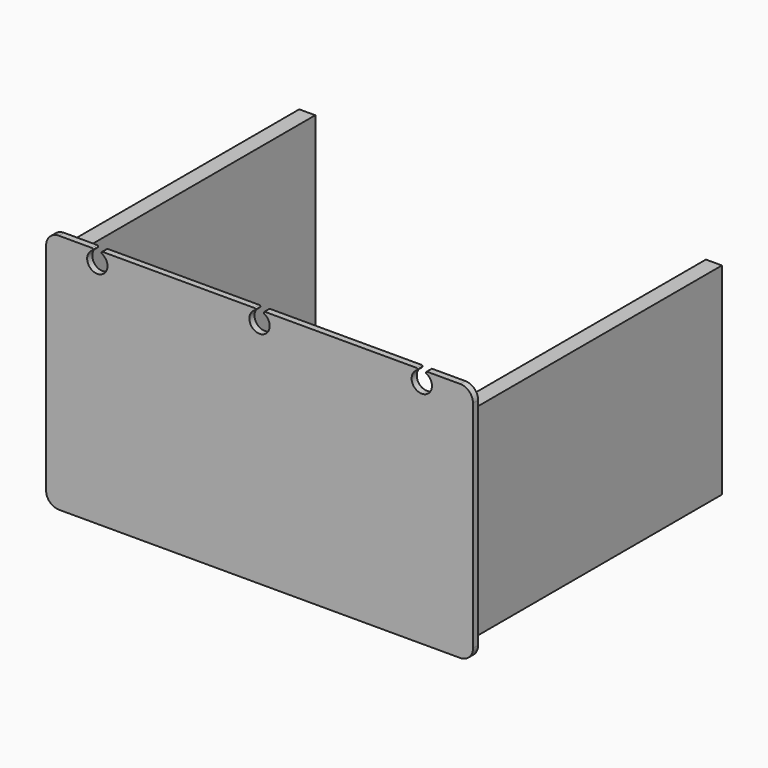
from build123d import *

# Parameters (mm, degrees)
F0_W     = 47.625
F0_H     = 600.075
F1_DEPTH = 914.4
F2_W     = 47.625
F2_H     = 600.075
F3_DEPTH = 19.05


# Not quite as in the source:
# - ends of sketch curves that miss each other by under 0.0002 mm in the source are joined


with BuildPart() as f1:
    # F0 (on Front) → F1 (new body)
    with BuildSketch(Plane.XZ):
        with Locations((-43.6453819275, 313.9032570556)):
            Rectangle(F0_W, F0_H)
    extrude(amount=F1_DEPTH)


with BuildPart() as f1b:
    # F0 (on Front) → F1, piece 2 (new body)
    with BuildSketch(Plane.XZ):
        with Locations((1166.0296180725, 313.9032570556)):
            Rectangle(F0_W, F0_H)
    extrude(amount=F1_DEPTH)

    # F2 (on face) → F3 (join)
    with BuildSketch(Plane.XZ.offset(914.4)):
        with BuildLine():
            Line((62.7171180725, 672.6782570556), (-35.7078819275, 672.6782570556))
            ThreePointArc((-35.7078819275, 672.6782570556), (-62.6486502907, 661.5190254188), (-73.8078819275, 634.5782570556))
            Line((-73.8078819275, 634.5782570556), (-73.8078819275, -6.7717429444))
            ThreePointArc((-73.8078819275, -6.7717429444), (-62.6486502907, -33.7125113076), (-35.7078819275, -44.8717429444))
            Line((-35.7078819275, -44.8717429444), (1158.0921180725, -44.8717429444))
            ThreePointArc((1158.0921180725, -44.8717429444), (1185.0328864357, -33.7125113076), (1196.1921180725, -6.7717429444))
            Line((1196.1921180725, -6.7717429444), (1196.1921180725, 634.5782570556))
            ThreePointArc((1196.1921180725, 634.5782570556), (1185.0328864357, 661.5190254188), (1158.0921180725, 672.6782570556))
            Line((1158.0921180725, 672.6782570556), (1059.6671180725, 672.6782570556))
            ThreePointArc((1059.6671180725, 672.6782570556), (1057.4220540422, 671.7483210859), (1056.4921180725, 669.5032570556))
            ThreePointArc((1056.4921180725, 669.5032570556), (1056.9402337169, 667.8769954804), (1058.1580876543, 666.7097910729))
            ThreePointArc((1058.1580876543, 666.7097910729), (1043.7921180725, 609.8899949171), (1029.4261484908, 666.7097910729))
            ThreePointArc((1029.4261484908, 666.7097910729), (1030.6440024281, 667.8769954804), (1031.0921180725, 669.5032570556))
            ThreePointArc((1031.0921180725, 669.5032570556), (1030.1621821028, 671.7483210859), (1027.9171180725, 672.6782570556))
            Line((1027.9171180725, 672.6782570556), (577.0670724869, 672.6782570556))
            ThreePointArc((577.0670724869, 672.6782570556), (574.8220084566, 671.7483210859), (573.8920724869, 669.5032570556))
            ThreePointArc((573.8920724869, 669.5032570556), (574.3401881312, 667.8769954804), (575.5580420686, 666.7097910729))
            ThreePointArc((575.5580420686, 666.7097910729), (561.1921180725, 609.8899949171), (546.8261484908, 666.7097910729))
            ThreePointArc((546.8261484908, 666.7097910729), (548.0439568425, 667.8769954804), (548.4920724869, 669.5032570556))
            ThreePointArc((548.4920724869, 669.5032570556), (547.5621365171, 671.7483210859), (545.3170724869, 672.6782570556))
            Line((545.3170724869, 672.6782570556), (94.4671180725, 672.6782570556))
            ThreePointArc((94.4671180725, 672.6782570556), (92.2220540422, 671.7483210859), (91.2921180725, 669.5032570556))
            ThreePointArc((91.2921180725, 669.5032570556), (91.7402337169, 667.8769954804), (92.9580876543, 666.7097910729))
            ThreePointArc((92.9580876543, 666.7097910729), (78.5921180725, 609.8899949171), (64.2261484908, 666.7097910729))
            ThreePointArc((64.2261484908, 666.7097910729), (65.4440024281, 667.8769954804), (65.8921180725, 669.5032570556))
            ThreePointArc((65.8921180725, 669.5032570556), (64.9621821028, 671.7483210859), (62.7171180725, 672.6782570556))
        make_face()
        with Locations((-43.6453819275, 313.9032570556)):
            Rectangle(F2_W, F2_H, mode=Mode.SUBTRACT)
        with Locations((-43.6453819275, 313.9032570556)):
            Rectangle(F2_W, F2_H)
    extrude(amount=F3_DEPTH)


solid = Compound([f1.part, f1b.part])
